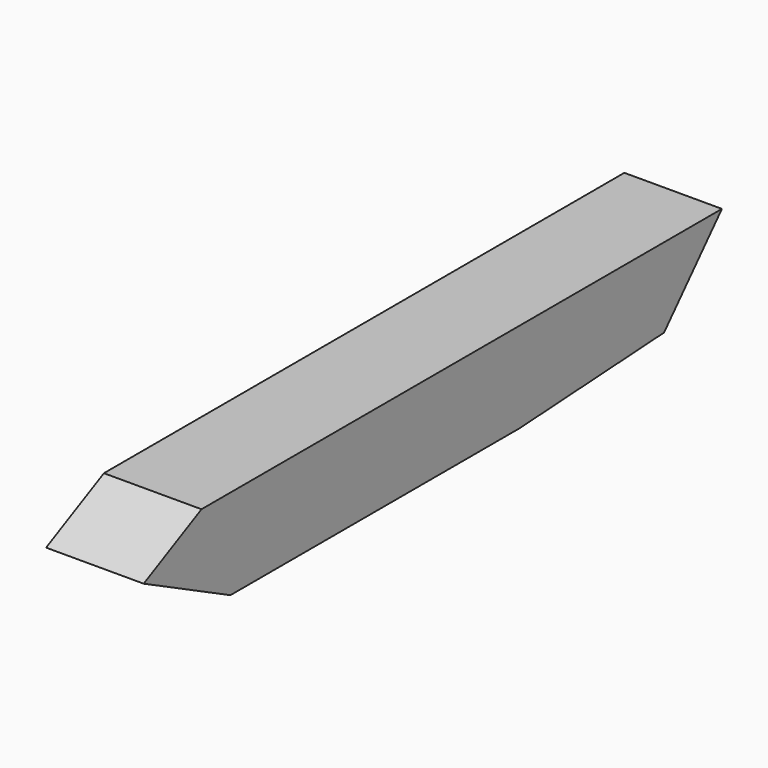
from build123d import *

# Parameters (mm, degrees)
F1_DEPTH = 27


# Not quite as in the source:
# - the program builds the solid bodies; features that only make, move or delete a surface that nothing else refers to are left out


with BuildPart() as f1:
    # F0 (on Right) → F1 (new body)
    with BuildSketch(Plane.YZ):
        Polygon((81.9772246434, 34.2262196874), (-98.0227753566, 34.2262196874), (-118.0227753566, 24.2262196874), (-88.0227753566, 9.2262196874), (11.9772246434, 9.2262196874), (61.9772246434, 12.2262196874), align=None)
    extrude(amount=F1_DEPTH)


solid = f1.part
